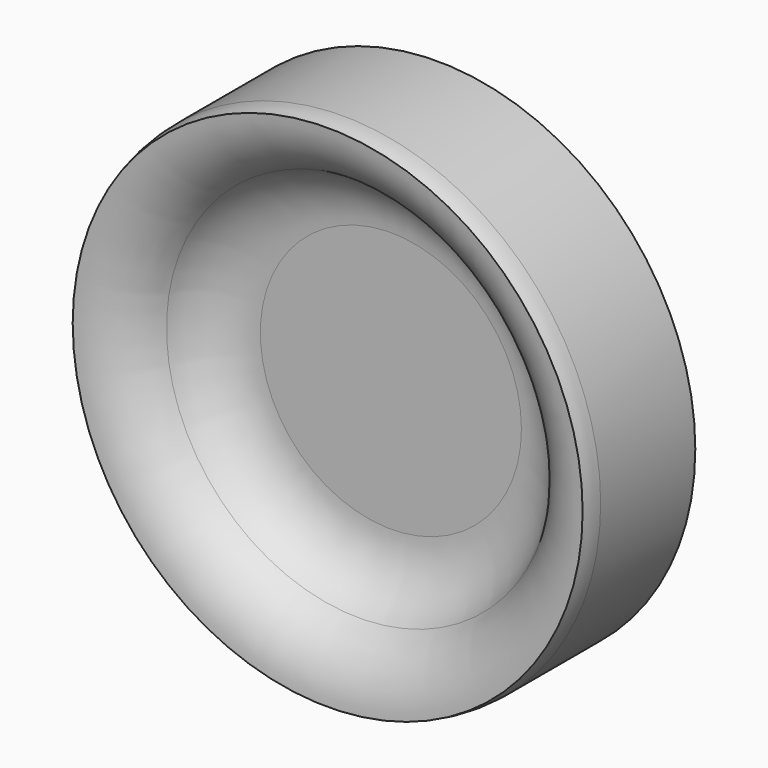
from build123d import *

# Parameters (mm, degrees)
F0_R     = 19.05
F1_DEPTH = 10.16
F2_T     = -4.318
F3_R     = 5.08


# Not quite as in the source:
# - a fillet or chamfer that OpenCascade refuses, or shapes differently, is made with other operations: its cross-section is extruded or revolved along the edge and cut away or added


with BuildPart() as f1:
    # F0 (on Front) → F1 (new body)
    with BuildSketch(Plane.XZ):
        Circle(F0_R)
    extrude(amount=F1_DEPTH)

    # F2
    f2_openings = [f1.faces().sort_by_distance(p)[0] for p in [
        (0, -10.16, 0),
    ]]
    offset(amount=F2_T, openings=f2_openings)

    # F3
    f3_edges = [f1.edges().sort_by_distance(p)[0] for p in [
        (-14.732, -4.318, 0),
    ]]
    fillet(f3_edges, radius=F3_R)

    # F4: fillet of radius 5.08 on 1 edges, made by hand

    # F4_s1 → F4_t2 (revolve, cut)
    with BuildSketch(Plane.XY):
        with BuildLine():
            ThreePointArc((14.2503822155, -7.239), (16.1249178862, -9.3680135261), (18.848764431, -10.16))
            Line((18.848764431, -10.16), (18.848764431, -10.668))
            Line((18.848764431, -10.668), (14.732, -10.668))
            Line((14.732, -10.668), (14.224, -10.16))
            ThreePointArc((14.224, -10.16), (14.224, -9.398), (13.790543994, -7.4549))
            Line((13.790543994, -7.4549), (14.2503822155, -7.239))
        make_face()
    revolve(axis=Axis((0, -10.16, 0), (0, -1, 0)), mode=Mode.SUBTRACT)

    # F5: fillet of radius 5.08 on 1 edges, made by hand

    # F5_s1 → F5_t2 (revolve, cut)
    with BuildSketch(Plane.XY):
        with BuildLine():
            ThreePointArc((18.848764431, -10.16), (18.9994394971, -9.4592919765), (19.05, -8.7443525768))
            Line((19.05, -8.7443525768), (19.05, -10.16))
            Line((19.05, -10.16), (18.848764431, -10.16))
        make_face()
    revolve(axis=Axis((0, -10.16, 0), (0, -1, 0)), mode=Mode.SUBTRACT)


solid = f1.part
